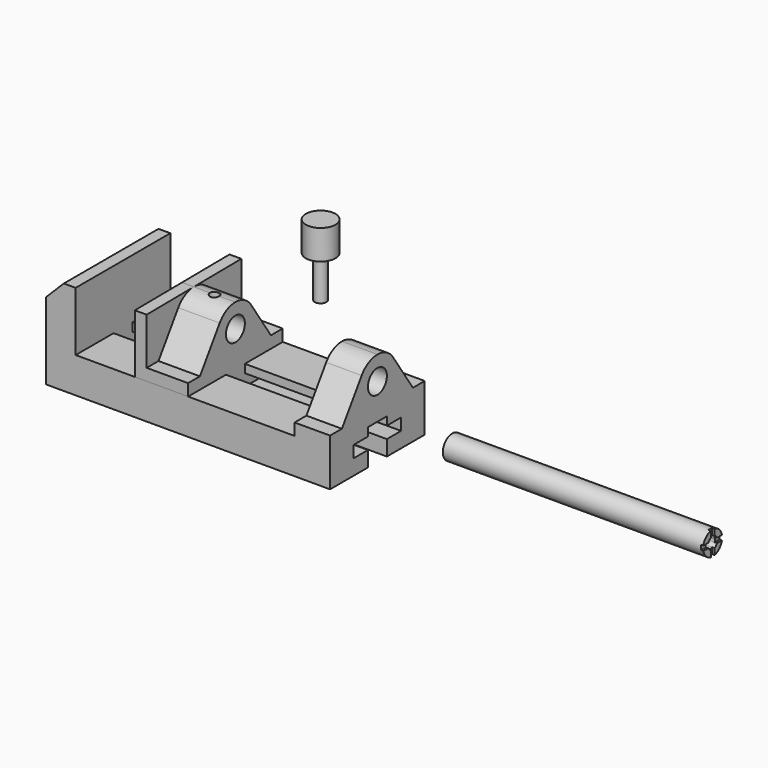
from build123d import *

# Parameters (mm, degrees)
F1_DEPTH  = 127
F3_DEPTH  = 273.05
F2_R      = 12.7
F4_DEPTH  = 38.1
F5_R      = 12.7
F6_DEPTH  = 57.15
F7_DEPTH  = 44.45
F8_R      = 5.08
F9_DEPTH  = 25.4
F10_R     = 12.7
F11_DEPTH = 279.4
F13_DEPTH = 25.4
F14_DEPTH = 2.54
F15_R     = 15.875
F16_DEPTH = 31.75
F17_R     = 6.35
F18_DEPTH = 44.45


with BuildPart() as f1:
    # F0 (on Front) → F1 (new body)
    with BuildSketch(Plane.XZ):
        Polygon((-152.4, 82.55), (-152.4, 0), (152.4, 0), (152.4, 101.6), (114.3, 101.6), (114.3, 38.1), (-120.65, 38.1), (-120.65, 101.6), (-133.35, 101.6), align=None)
    extrude(amount=F1_DEPTH)

    # F2 (on face) → F3 (cut, through all)
    with BuildSketch(Plane.YZ.offset(152.4)):
        Polygon((-76.2, 16.51), (-76.2, 0), (-50.8, 0), (-50.8, 16.51), (-31.75, 16.51), (-31.75, 29.21), (-50.8, 29.21), (-50.8, 38.1), (-76.2, 38.1), (-76.2, 29.21), (-95.25, 29.21), (-95.25, 16.51), align=None)
    extrude(amount=-F3_DEPTH, mode=Mode.SUBTRACT)

    # F2 (on face) → F4 (cut, through all)
    with BuildSketch(Plane.YZ.offset(152.4)):
        with BuildLine():
            Line((-127, 101.6), (-127, 50.8))
            Line((-127, 50.8), (-111.125, 50.8))
            Line((-111.125, 50.8), (-84.5934256055, 90.3501730104))
            ThreePointArc((-84.5934256055, 90.3501730104), (-75.4529411765, 98.6117647059), (-63.5, 101.6))
            Line((-63.5, 101.6), (-127, 101.6))
        make_face()
        with BuildLine():
            Line((0, 101.6), (-63.5, 101.6))
            ThreePointArc((-63.5, 101.6), (-51.5470588235, 98.6117647059), (-42.4065743945, 90.3501730104))
            Line((-42.4065743945, 90.3501730104), (-15.875, 50.8))
            Line((-15.875, 50.8), (0, 50.8))
            Line((0, 50.8), (0, 101.6))
        make_face()
        with Locations((-63.5, 76.2)):
            Circle(F2_R)
    extrude(amount=-F4_DEPTH, mode=Mode.SUBTRACT)


with BuildPart() as f6:
    # F5 (on Right) → F6 (new body)
    with BuildSketch(Plane.YZ):
        with BuildLine():
            Line((-95.25, 29.21), (-95.25, 16.51))
            Line((-95.25, 16.51), (-31.75, 16.51))
            Line((-31.75, 16.51), (-31.75, 29.21))
            Line((-31.75, 29.21), (-50.8, 29.21))
            Line((-50.8, 29.21), (-50.8, 38.1))
            Line((-50.8, 38.1), (0, 38.1))
            Line((0, 38.1), (0, 50.8))
            Line((0, 50.8), (-15.875, 50.8))
            Line((-15.875, 50.8), (-42.4065743945, 90.3501730104))
            ThreePointArc((-42.4065743945, 90.3501730104), (-51.6500867545, 98.6664095056), (-63.7332419371, 101.5989290758))
            ThreePointArc((-63.7332419371, 101.5989290758), (-75.555717124, 98.5566474371), (-84.5934256055, 90.3501730104))
            Line((-84.5934256055, 90.3501730104), (-111.125, 50.8))
            Line((-111.125, 50.8), (-127, 50.8))
            Line((-127, 50.8), (-127, 38.1))
            Line((-127, 38.1), (-76.2, 38.1))
            Line((-76.2, 38.1), (-76.2, 29.21))
            Line((-76.2, 29.21), (-95.25, 29.21))
        make_face()
        with Locations((-63.5, 76.2)):
            Circle(F5_R, mode=Mode.SUBTRACT)
        with BuildLine():
            Line((-127, 101.0179419357), (-127, 50.8))
            Line((-127, 50.8), (-111.125, 50.8))
            Line((-111.125, 50.8), (-84.5934256055, 90.3501730104))
            ThreePointArc((-84.5934256055, 90.3501730104), (-75.555717124, 98.5566474371), (-63.7332419371, 101.5989290758))
            Line((-63.7332419371, 101.5989290758), (-127, 101.0179419357))
        make_face()
        with BuildLine():
            Line((-15.875, 50.8), (0, 50.8))
            Line((0, 50.8), (0, 102.1842))
            Line((0, 102.1842), (-63.5, 101.6010709679))
            Line((-63.5, 101.6010709679), (-63.7332419371, 101.5989290758))
            ThreePointArc((-63.7332419371, 101.5989290758), (-51.6500867545, 98.6664095056), (-42.4065743945, 90.3501730104))
            Line((-42.4065743945, 90.3501730104), (-15.875, 50.8))
        make_face()
    extrude(amount=-F6_DEPTH)

    # F5 (on Right) → F7 (cut)
    with BuildSketch(Plane.YZ):
        with BuildLine():
            Line((-127, 101.0179419357), (-127, 50.8))
            Line((-127, 50.8), (-111.125, 50.8))
            Line((-111.125, 50.8), (-84.5934256055, 90.3501730104))
            ThreePointArc((-84.5934256055, 90.3501730104), (-75.555717124, 98.5566474371), (-63.7332419371, 101.5989290758))
            Line((-63.7332419371, 101.5989290758), (-127, 101.0179419357))
        make_face()
        with BuildLine():
            Line((-15.875, 50.8), (0, 50.8))
            Line((0, 50.8), (0, 102.1842))
            Line((0, 102.1842), (-63.5, 101.6010709679))
            Line((-63.5, 101.6010709679), (-63.7332419371, 101.5989290758))
            ThreePointArc((-63.7332419371, 101.5989290758), (-51.6500867545, 98.6664095056), (-42.4065743945, 90.3501730104))
            Line((-42.4065743945, 90.3501730104), (-15.875, 50.8))
        make_face()
    extrude(amount=-F7_DEPTH, mode=Mode.SUBTRACT)

    # F8 (on face) → F9 (cut)
    with BuildSketch(Plane(origin=(0, -0.9382921124, 102.1755835375), x_dir=(1, 0, 0), z_dir=(0, -0.0091827472, 0.9999578377))):
        with Locations((-22.225, -62.5616683254)):
            Circle(F8_R)
    extrude(amount=-F9_DEPTH, mode=Mode.SUBTRACT)


with BuildPart() as f11:
    # F10 (on face) → F11 (new body)
    with BuildSketch(Plane.YZ.offset(152.4)):
        with Locations((37.0000302792, -26.4865104109)):
            Circle(F10_R)
    extrude(amount=F11_DEPTH)

    # F12 (on face) → F13 (cut)
    with BuildSketch(Plane.YZ.offset(431.8)):
        with BuildLine():
            ThreePointArc((42.8199014118, -29.0265104109), (43.2160853663, -27.7838766483), (43.3500302792, -26.4865104109))
            ThreePointArc((43.3500302792, -26.4865104109), (43.2160853663, -25.1891441735), (42.8199014118, -23.9465104109))
            ThreePointArc((42.8199014118, -23.9465104109), (41.4901583397, -21.9963823504), (39.5400302792, -20.6666392783))
            ThreePointArc((39.5400302792, -20.6666392783), (37.0000302792, -20.1365104109), (34.4600302792, -20.6666392783))
            ThreePointArc((34.4600302792, -20.6666392783), (32.5099022186, -21.9963823504), (31.1801591466, -23.9465104109))
            ThreePointArc((31.1801591466, -23.9465104109), (30.6500302792, -26.4865104109), (31.1801591466, -29.0265104109))
            ThreePointArc((31.1801591466, -29.0265104109), (32.5099022186, -30.9766384714), (34.4600302792, -32.3063815435))
            ThreePointArc((34.4600302792, -32.3063815435), (37.0000302792, -32.8365104109), (39.5400302792, -32.3063815435))
            ThreePointArc((39.5400302792, -32.3063815435), (41.4901583397, -30.9766384714), (42.8199014118, -29.0265104109))
        make_face()
    extrude(amount=-F13_DEPTH, mode=Mode.SUBTRACT)

    # F12 (on face) → F14 (cut)
    with BuildSketch(Plane.YZ.offset(431.8)):
        with BuildLine():
            ThreePointArc((31.1801591466, -29.0265104109), (30.6500302792, -26.4865104109), (31.1801591466, -23.9465104109))
            Line((31.1801591466, -23.9465104109), (24.5566223858, -23.9465104109))
            ThreePointArc((24.5566223858, -23.9465104109), (24.3000302792, -26.4865104109), (24.5566223858, -29.0265104109))
            Line((24.5566223858, -29.0265104109), (31.1801591466, -29.0265104109))
        make_face()
        with BuildLine():
            ThreePointArc((34.4600302792, -20.6666392783), (37.0000302792, -20.1365104109), (39.5400302792, -20.6666392783))
            Line((39.5400302792, -20.6666392783), (39.5400302792, -14.0431025176))
            ThreePointArc((39.5400302792, -14.0431025176), (37.0000302792, -13.7865104109), (34.4600302792, -14.0431025176))
            Line((34.4600302792, -14.0431025176), (34.4600302792, -20.6666392783))
        make_face()
        with BuildLine():
            ThreePointArc((42.8199014118, -23.9465104109), (43.2160853663, -25.1891441735), (43.3500302792, -26.4865104109))
            ThreePointArc((43.3500302792, -26.4865104109), (43.2160853663, -27.7838766483), (42.8199014118, -29.0265104109))
            Line((42.8199014118, -29.0265104109), (49.4434381725, -29.0265104109))
            ThreePointArc((49.4434381725, -29.0265104109), (49.6357194223, -27.7629742284), (49.7000302792, -26.4865104109))
            ThreePointArc((49.7000302792, -26.4865104109), (49.6357194223, -25.2100465934), (49.4434381725, -23.9465104109))
            Line((49.4434381725, -23.9465104109), (42.8199014118, -23.9465104109))
        make_face()
        with BuildLine():
            Line((39.5400302792, -38.9299183042), (39.5400302792, -32.3063815435))
            ThreePointArc((39.5400302792, -32.3063815435), (37.0000302792, -32.8365104109), (34.4600302792, -32.3063815435))
            Line((34.4600302792, -32.3063815435), (34.4600302792, -38.9299183042))
            ThreePointArc((34.4600302792, -38.9299183042), (37.0000302792, -39.1865104109), (39.5400302792, -38.9299183042))
        make_face()
    extrude(amount=-F14_DEPTH, mode=Mode.SUBTRACT)


with BuildPart() as f16:
    # F15 (on face) → F16 (new body)
    with BuildSketch(Plane.XY.offset(101.6)):
        with Locations((0, 50.8)):
            Circle(F15_R)
    extrude(amount=F16_DEPTH)

    # F17 (on face) → F18 (join)
    with BuildSketch(Plane(origin=(0, 0, 101.6), x_dir=(1, 0, 0), z_dir=(0, 0, -1))):
        with Locations((0, -50.8)):
            Circle(F17_R)
    extrude(amount=F18_DEPTH)


solid = Compound([f1.part, f6.part, f11.part, f16.part])
